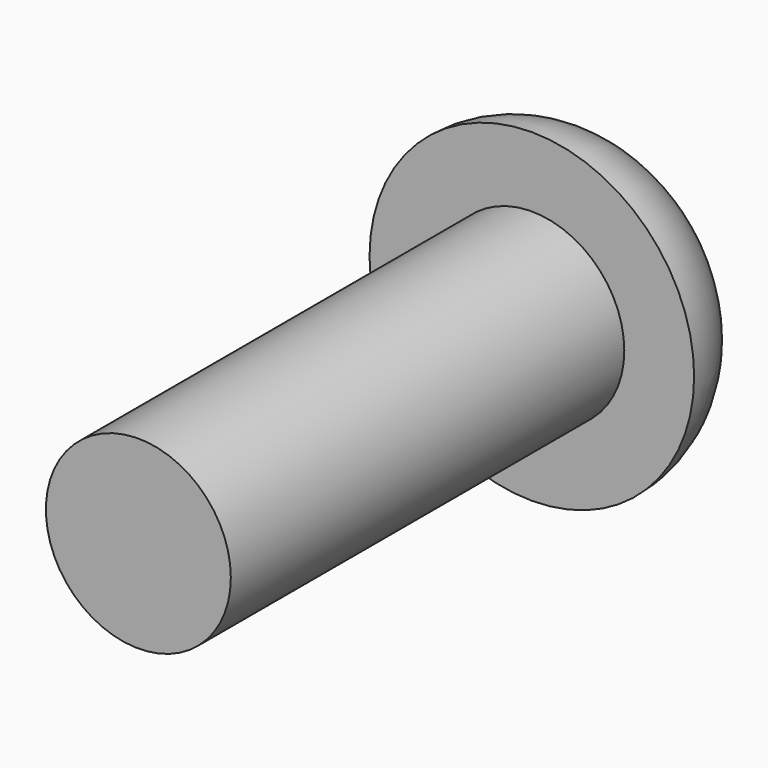
from build123d import *

# Parameters (mm, degrees)
F0_R     = 4.191
F1_DEPTH = 2.5654
F2_R     = 2.3876
F3_DEPTH = 12.7
F5_DEPTH = 1.27


# Not quite as in the source:
# - a fillet or chamfer that OpenCascade refuses, or shapes differently, is made with other operations: its cross-section is extruded or revolved along the edge and cut away or added


with BuildPart() as f1:
    # F0 (on Front) → F1 (new body)
    with BuildSketch(Plane.XZ):
        Circle(F0_R)
    extrude(amount=-F1_DEPTH)

    # F2 (on face) → F3 (join)
    with BuildSketch(Plane.XZ):
        Circle(F2_R)
    extrude(amount=F3_DEPTH)

    # F4 (on face) → F5 (cut)
    with BuildSketch(Plane(origin=(0, 2.5654, 0), x_dir=(-1, 0, 0), z_dir=(0, 1, 0))):
        Polygon((-2.3449476001, 0.0811547043), (-1.2427558356, -1.9902068401), (1.1021917645, -2.0713615444), (2.3449476001, -0.0811547043), (1.2427558356, 1.9902068401), (-1.1021917645, 2.0713615444), align=None)
    extrude(amount=-F5_DEPTH, mode=Mode.SUBTRACT)

    # F6: fillet of radius 2.5654 on 1 edges, made by hand

    # F6_s1 → F6_t2 (revolve, cut)
    with BuildSketch(Plane.XY):
        with BuildLine():
            ThreePointArc((4.191, 0), (3.4396117365, 1.8140117365), (1.6256, 2.5654))
            Line((1.6256, 2.5654), (4.191, 2.5654))
            Line((4.191, 2.5654), (4.191, 0))
        make_face()
    revolve(axis=Axis((0, 2.5654, 0), (0, -1, 0)), mode=Mode.SUBTRACT)


solid = f1.part
